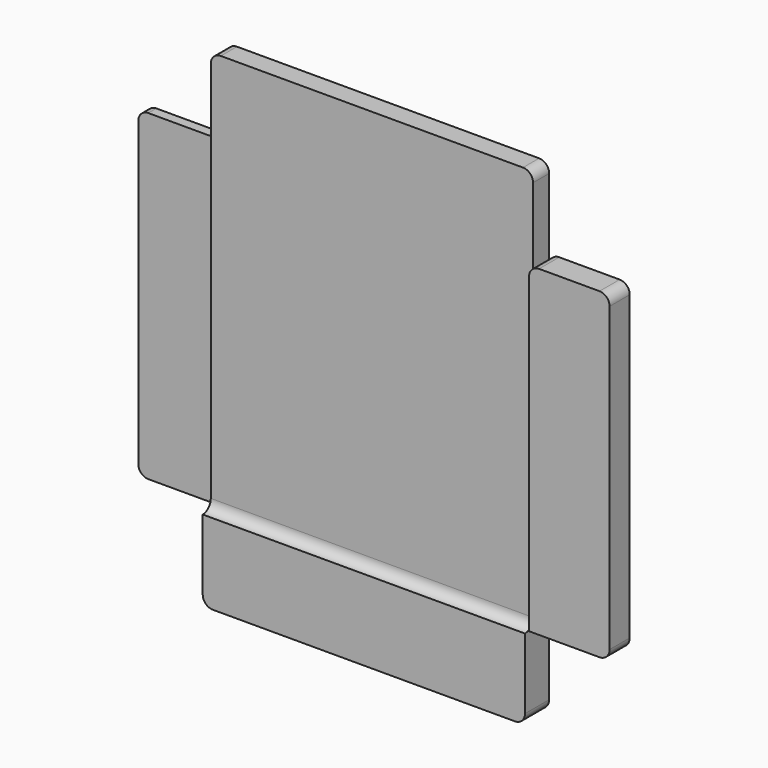
from build123d import *

# Parameters (mm, degrees)
F0_W     = 50.8
F0_H     = 12.7
F1_DEPTH = 3.175
F0_W_2   = 12.7
F0_H_2   = 50.8
F2_DEPTH = 3.96875
F3_DEPTH = 4.7625
F4_DEPTH = 1.5875
F5_DEPTH = 3.175
F6_R     = 1.58749
F6_2_R   = 1.58749


# Not quite as in the source:
# - a fillet or chamfer is up to 0.001 mm smaller than in the source, because OpenCascade refuses the exact size


with BuildPart() as f1:
    # F0 (on Front) → F1 (new body)
    with BuildSketch(Plane.XZ):
        with Locations((0, 31.75)):
            Rectangle(F0_W, F0_H)
    extrude(amount=F1_DEPTH)



with BuildPart() as f2:
    # F0 (on Front) → F2 (new body)
    with BuildSketch(Plane.XZ):
        with Locations((31.75, 0)):
            Rectangle(F0_W_2, F0_H_2)
    extrude(amount=F2_DEPTH)

    # F6#2 (radius 1.5875 in the source; OpenCascade refuses exactly that, so slightly less here)
    f6_2_edges = [f2.edges().sort_by_distance(p)[0] for p in [
        (38.1, -1.984375, -25.4),
        (25.4, -1.984375, 25.4),
        (38.1, -1.984375, 25.4),
    ]]
    fillet(f6_2_edges, radius=F6_2_R)


with BuildPart() as f3:
    # F0 (on Front) → F3 (new body)
    with BuildSketch(Plane.XZ):
        with Locations((0, -31.75)):
            Rectangle(F0_W, F0_H)
    extrude(amount=F3_DEPTH)


with BuildPart() as f1_1:
    add(f1.part)

    add(f3.part)  # F4 merges F3
    # F0 (on Front) → F4 (join)
    with BuildSketch(Plane.XZ):
        with Locations((-31.75, 0)):
            Rectangle(F0_W_2, F0_H_2)
    extrude(amount=F4_DEPTH)

    # F0 (on Front) → F5 (join)
    with BuildSketch(Plane.XZ):
        Rectangle(F0_W, F0_H_2)
    extrude(amount=F5_DEPTH)

    # F6 (radius 1.5875 in the source; OpenCascade refuses exactly that, so slightly less here)
    f6_edges = [f1_1.edges().sort_by_distance(p)[0] for p in [
        (-25.4, -2.38125, -38.1),
        (25.4, -2.38125, -38.1),
        (-38.1, -0.79375, -25.4),
        (-38.1, -0.79375, 25.4),
        (-25.4, -0.79375, 25.4),
        (-25.4, -1.5875, 38.1),
        (25.4, -1.5875, 38.1),
        (-25.4, -0.79375, -25.4),
        (0, -3.175, -25.4),
    ]]
    fillet(f6_edges, radius=F6_R)


solid = Compound([f2.part, f1_1.part])
